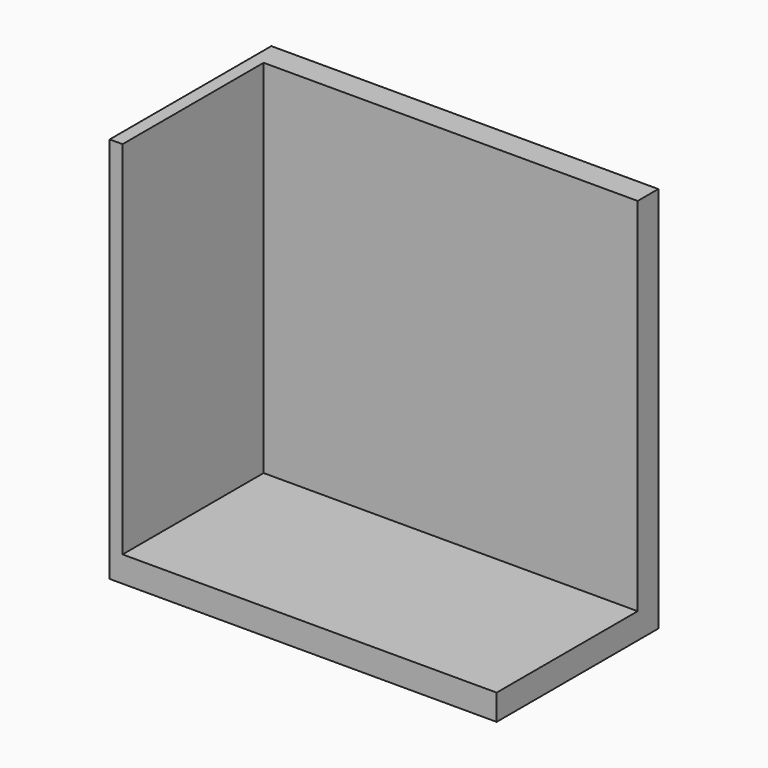
from build123d import *

# Parameters (mm, degrees)
F1_DEPTH = 90
F3_W     = 47
F3_H     = 90
F4_DEPTH = 3


# Not quite as in the source:
# - the program builds the solid bodies; features that only make, move or delete a surface that nothing else refers to are left out


with BuildPart() as f1:
    # F0 (on Right) → F1 (new body)
    with BuildSketch(Plane.YZ):
        Polygon((47, 0), (47, 90), (41, 90), (41, 6), (0, 6), (0, 0), align=None)
    extrude(amount=F1_DEPTH)

    # F3 (on face) → F4 (join)
    with BuildSketch(Plane(origin=(0, 0, 0), x_dir=(0, -1, 0), z_dir=(-1, 0, 0))):
        with Locations((-23.5, 45)):
            Rectangle(F3_W, F3_H)
    extrude(amount=-F4_DEPTH)


solid = f1.part
